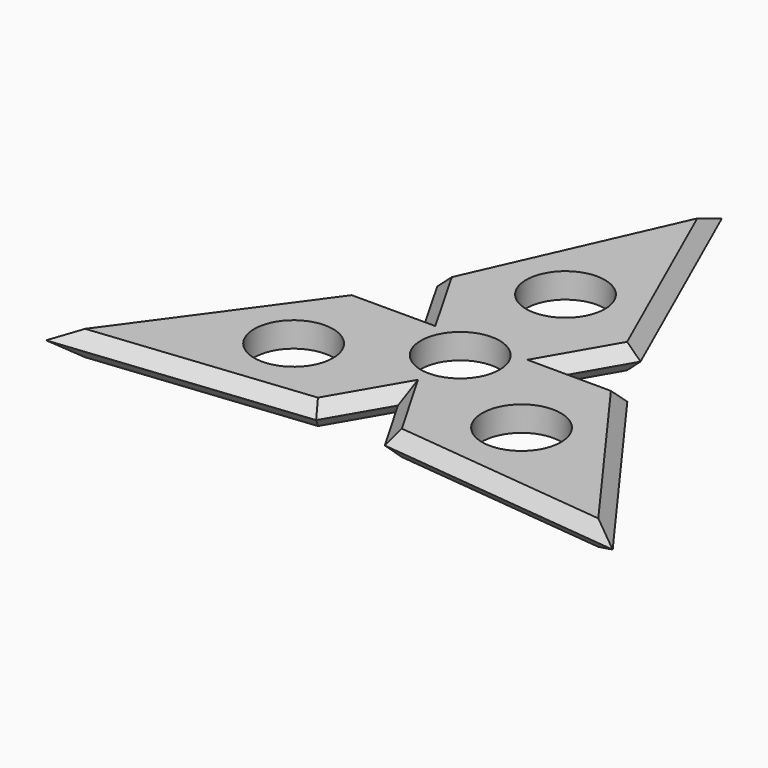
from build123d import *

# Parameters (mm, degrees)
F0_R     = 11
F1_DEPTH = 7
F2_SIZE  = 3.49999


# Not quite as in the source:
# - a fillet or chamfer is up to 0.001 mm smaller than in the source, because OpenCascade refuses the exact size


with BuildPart() as f1:
    # F0 (on Top) → F1 (new body)
    with BuildSketch(Plane.XY):
        Polygon((28.3908957982, 27.4554844946), (0, 91.3447894481), (-28.3908957982, 27.4554844946), (-18.890943275, 10.8594947502), (-37.9725949446, 10.8594947502), (-79.1069081654, -45.6723947241), (-9.5816991464, -38.3149792447), (0.0408733116, -21.7897841527), (9.5816991464, -38.3149792447), (79.1069081654, -45.6723947241), (37.9725949446, 10.8594947502), (18.8500699634, 10.9302894025), align=None)
        with Locations((-31.8169734902, -18.3695382094)):
            Circle(F0_R, mode=Mode.SUBTRACT)
        with Locations((31.8169734902, -18.3695382094)):
            Circle(F0_R, mode=Mode.SUBTRACT)
        Circle(F0_R, mode=Mode.SUBTRACT)
        with Locations((0, 36.7390764187)):
            Circle(F0_R, mode=Mode.SUBTRACT)
    extrude(amount=F1_DEPTH)

    # F2 (size 3.5 in the source; OpenCascade refuses exactly that, so slightly less here)
    f2_edges = [f1.edges().sort_by_distance(p)[0] for p in [
        (-44.344304, -41.993687, 7),
        (-4.770413, -30.052382, 0),
        (-44.344304, -41.993687, 0),
        (-4.770413, -30.052382, 7),
        (4.811286, -30.052382, 7),
        (4.811286, -30.052382, 0),
        (44.344304, -41.993687, 7),
        (44.344304, -41.993687, 0),
        (-58.539752, -17.40645, 7),
        (58.539752, -17.40645, 7),
        (-14.195448, 59.400137, 7),
        (14.195448, 59.400137, 7),
        (-28.431769, 10.859495, 7),
        (-23.64092, 19.15749, 7),
        (23.620483, 19.192887, 0),
        (28.411332, 10.894892, 7),
        (23.620483, 19.192887, 7),
        (-28.431769, 10.859495, 0),
        (-58.539752, -17.40645, 0),
        (-14.195448, 59.400137, 0),
        (14.195448, 59.400137, 0),
        (58.539752, -17.40645, 0),
        (28.411332, 10.894892, 0),
    ]]
    chamfer(f2_edges, length=F2_SIZE)


solid = f1.part
